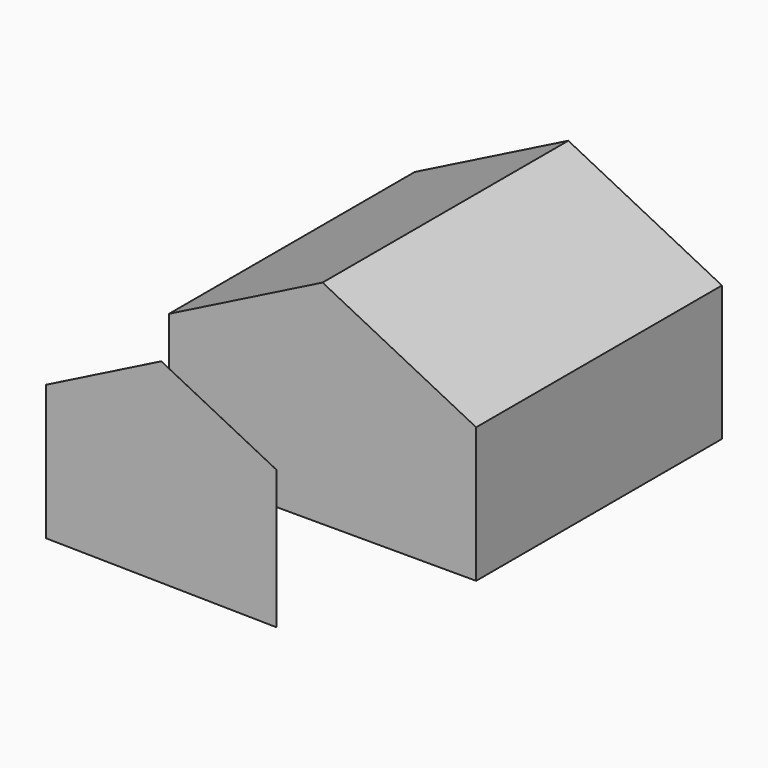
from build123d import *

# Parameters (mm, degrees)
F0_W     = 127000
F0_H     = 55880
F1_DEPTH = 127000
F3_DEPTH = 127000
F8_DEPTH = 25.4


# Not quite as in the source:
# - the program builds the solid bodies; features that only make, move or delete a surface that nothing else refers to are left out


with BuildPart() as f1:
    # F0 (on Front) → F1 (new body)
    with BuildSketch(Plane.XZ):
        Rectangle(F0_W, F0_H)
    extrude(amount=F1_DEPTH)

    # F2 (on face) → F3 (join)
    with BuildSketch(Plane.XZ.offset(127000)):
        Polygon((0, 59968.181340813), (-63500, 27940), (63500, 27940), align=None)
    extrude(amount=-F3_DEPTH)


with BuildPart() as f8:
    # F7 (on offset) → F8 (new body)
    with BuildSketch(Plane.XZ.offset(190500)):
        Polygon((-15875, 51961.1360056098), (-63500, 27940), (-63500, -27940), (31750, -29356.3232421875), (31750, 27940), align=None)
    extrude(amount=-F8_DEPTH)


solid = Compound([f1.part, f8.part])
